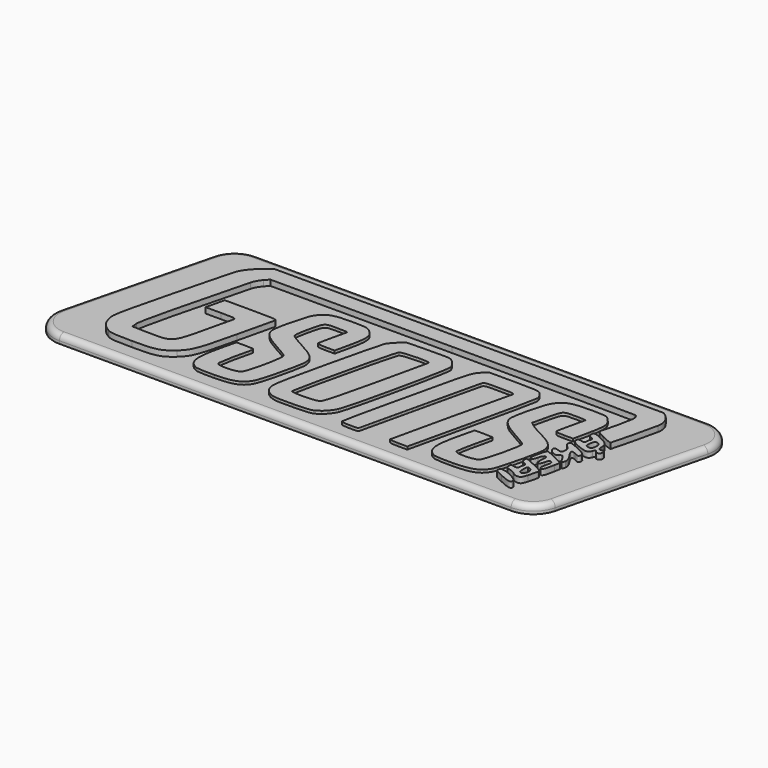
from build123d import *

# Parameters (mm, degrees)
F1_DEPTH = 3
F3_DEPTH = 2
F5_DEPTH = 1
F6_R     = 10
F7_R     = 2


# Not quite as in the source:
# - ends of sketch curves that miss each other by under 0.0002 mm in the source are joined


with BuildPart() as f1:
    # F0 (on Top) → F1 (new body)
    with BuildSketch(Plane.XY):
        Polygon((100, 36), (-82.0483837953, 36), (-100, -36), (82.0483837953, -36), align=None)
    extrude(amount=-F1_DEPTH)

    # F6
    f6_edges = [f1.edges().sort_by_distance(p)[0] for p in [
        (82.048384, -36, -1.5),
        (100, 36, -1.5),
        (-82.048384, 36, -1.5),
        (-100, -36, -1.5),
    ]]
    fillet(f6_edges, radius=F6_R)

    # F7
    f7_edges = [f1.edges().sort_by_distance(p)[0] for p in [
        (90.421013, -2.419219, 0),
        (80.392142, -33.880108, 0),
        (95.080691, 32.156615, 0),
        (-6.482528, -36, 0),
        (6.482528, 36, 0),
        (-95.080691, -32.156615, 0),
        (-80.392142, 33.880108, 0),
        (-90.421013, 2.419219, 0),
    ]]
    fillet(f7_edges, radius=F7_R)


with BuildPart() as f3:
    # F2 (on Top) → F3 (new body)
    with BuildSketch(Plane.XY):
        with BuildLine():
            add(Edge.make_bspline(
                [(-75.795616532, -28.4242405015), (-78.2587663788, -26.9027705255), (-79.2517103888, -25.5686924543), (-79.9744679458, -22.8097125669)],
                knots=[0, 0, 0, 0, 1, 1, 1, 1], degree=3))
            add(Edge.make_bspline(
                [(-66.5146440238, -29.4511190722), (-72.9671780187, -29.4493452772), (-74.3910725204, -29.2918230737), (-75.795616532, -28.4242405015)],
                knots=[0, 0, 0, 0, 1, 1, 1, 1], degree=3))
            add(Edge.make_bspline(
                [(-53.1869458343, -26.1183050096), (-56.5493552568, -29.0705405866), (-58.0804062385, -29.4534059483), (-66.5146440238, -29.4511190722)],
                knots=[0, 0, 0, 0, 1, 1, 1, 1], degree=3))
            add(Edge.make_bspline(
                [(-46.1866547532, -8.0317014306), (-49.2081877021, -21.146458367), (-50.0749640039, -23.3859446112), (-53.1869458343, -26.1183050096)],
                knots=[0, 0, 0, 0, 1, 1, 1, 1], degree=3))
            add(Edge.make_bspline(
                [(-43.1147267619, 4.9727765604), (-43.2790551442, 4.4404873009), (-44.6614235781, -1.4115239207), (-46.1866547532, -8.0317014306)],
                knots=[0, 0, 0, 0, 1, 1, 1, 1], degree=3))
            add(Edge.make_bspline(
                [(-52.2441455618, 5.9405733101), (-43.5197760782, 5.9405733101), (-42.8382534939, 5.8683272922), (-43.1147267619, 4.9727765604)],
                knots=[0, 0, 0, 0, 1, 1, 1, 1], degree=3))
            Line((-52.2441455618, 5.9405733101), (-61.6723430484, 5.9405733101))
            Line((-61.6723430484, 5.9405733101), (-62.0130645506, 4.4197483504))
            add(Edge.make_bspline(
                [(-62.8085644531, 1.1015853731), (-62.5584384271, 2.0901231676), (-62.200462738, 3.583294099), (-62.0130645506, 4.4197483504)],
                knots=[0, 0, 0, 0, 1, 1, 1, 1], degree=3))
            Line((-62.8085644531, 1.1015853731), (-63.2633428535, -0.6957547387))
            Line((-63.2633428535, -0.6957547387), (-57.7403800137, -0.6957547387))
            add(Edge.make_bspline(
                [(-52.5163382668, -1.6635535826), (-52.2454397829, -0.7864905268), (-52.7352228847, -0.6957547387), (-57.7403800137, -0.6957547387)],
                knots=[0, 0, 0, 0, 1, 1, 1, 1], degree=3))
            add(Edge.make_bspline(
                [(-54.5073906057, -10.0972238374), (-53.5767178968, -5.9909912107), (-52.6807441349, -2.195842842), (-52.5163382668, -1.6635535826)],
                knots=[0, 0, 0, 0, 1, 1, 1, 1], degree=3))
            add(Edge.make_bspline(
                [(-65.8975644353, -22.6981373061), (-57.4239911245, -22.9199936065), (-57.410200759, -22.9047331064), (-54.5073906057, -10.0972238374)],
                knots=[0, 0, 0, 0, 1, 1, 1, 1], degree=3))
            Line((-65.8975644353, -22.6981373061), (-71.9244253447, -22.540338667))
            Line((-71.9244253447, -22.540338667), (-72.0935473713, -20.508711031))
            add(Edge.make_bspline(
                [(-62.7643180079, 18.7170547803), (-69.3169468103, -6.5522517558), (-72.2342572659, -18.8184059351), (-72.0935473713, -20.508711031)],
                knots=[0, 0, 0, 0, 1, 1, 1, 1], degree=3))
            add(Edge.make_bspline(
                [(-60.8908869106, 22.1734774279), (-61.637107984, 21.3682897151), (-62.4801527107, 19.8128998378), (-62.7643180079, 18.7170547803)],
                knots=[0, 0, 0, 0, 1, 1, 1, 1], degree=3))
            Line((-60.8908869106, 22.1734774279), (-59.5341201804, 23.6374508991))
            Line((-59.5341201804, 23.6374508991), (5.4277806453, 23.6374508991))
            add(Edge.make_bspline(
                [(71.2644555565, 23.3017701577), (70.7833320084, 23.4863956126), (41.1568291361, 23.6374508991), (5.4277806453, 23.6374508991)],
                knots=[0, 0, 0, 0, 1, 1, 1, 1], degree=3))
            add(Edge.make_bspline(
                [(72.1392317362, 21.3200621788), (72.1392317362, 22.3108617188), (71.7910129663, 23.0997125082), (71.2644555565, 23.3017701577)],
                knots=[0, 0, 0, 0, 1, 1, 1, 1], degree=3))
            add(Edge.make_bspline(
                [(69.6190942774, 9.7772665945), (70.7649155355, 13.6800761474), (72.1392317362, 19.974729829), (72.1392317362, 21.3200621788)],
                knots=[0, 0, 0, 0, 1, 1, 1, 1], degree=3))
            add(Edge.make_bspline(
                [(72.6814852415, 7.3282945418), (70.3223694092, 8.4558480159), (69.4386279213, 9.1625681214), (69.6190942774, 9.7772665945)],
                knots=[0, 0, 0, 0, 1, 1, 1, 1], degree=3))
            add(Edge.make_bspline(
                [(76.2098251162, 5.9802208726), (76.0930708769, 5.8499443266), (74.5053170956, 6.4565800955), (72.6814852415, 7.3282945418)],
                knots=[0, 0, 0, 0, 1, 1, 1, 1], degree=3))
            add(Edge.make_bspline(
                [(80.150160798, 22.3358519134), (79.4319309206, 18.7363340673), (76.4135476618, 6.2075367755), (76.2098251162, 5.9802208726)],
                knots=[0, 0, 0, 0, 1, 1, 1, 1], degree=3))
            add(Edge.make_bspline(
                [(76.4670232856, 29.2734046848), (79.2593031884, 27.7829583192), (80.6967765404, 25.0753326219), (80.150160798, 22.3358519134)],
                knots=[0, 0, 0, 0, 1, 1, 1, 1], degree=3))
            Line((76.4670232856, 29.2734046848), (-62.5478145054, 29.3525971936))
            add(Edge.make_bspline(
                [(-69.849839202, 21.7018573997), (-68.9301925028, 24.02660517), (-65.2045907169, 27.9301246598), (-62.5478145054, 29.3525971936)],
                knots=[0, 0, 0, 0, 1, 1, 1, 1], degree=3))
            add(Edge.make_bspline(
                [(-75.5653436062, -0.1427265287), (-72.7827913036, 10.9593009126), (-70.2108137982, 20.7893624239), (-69.849839202, 21.7018573997)],
                knots=[0, 0, 0, 0, 1, 1, 1, 1], degree=3))
            add(Edge.make_bspline(
                [(-79.9744679458, -22.8097125669), (-80.5884837068, -20.4658383868), (-80.3439806317, -19.2088669923), (-75.5653436062, -0.1427265287)],
                knots=[0, 0, 0, 0, 1, 1, 1, 1], degree=3))
        make_face()
    extrude(amount=F3_DEPTH)


with BuildPart() as f3b:
    # F2 (on Top) → F3, piece 2 (new body)
    with BuildSketch(Plane.XY):
        with BuildLine():
            add(Edge.make_bspline(
                [(70.3418895302, -1.1602418914), (68.5422039045, -0.3665325375), (67.715012339, 0.3276872352), (67.715012339, 1.0443673981)],
                knots=[0, 0, 0, 0, 1, 1, 1, 1], degree=3))
            add(Edge.make_bspline(
                [(75.3841413811, -1.1542315119), (74.8334628735, -2.6428580101), (73.7066716914, -2.644200398), (70.3418895302, -1.1602418914)],
                knots=[0, 0, 0, 0, 1, 1, 1, 1], degree=3))
            add(Edge.make_bspline(
                [(76.228501271, -0.6012012077), (75.9633053179, -0.1721061851), (75.6784279897, -0.3586960078), (75.3841413811, -1.1542315119)],
                knots=[0, 0, 0, 0, 1, 1, 1, 1], degree=3))
            add(Edge.make_bspline(
                [(78.222531575, -0.0782269894), (78.222531575, -1.3307419074), (76.8946230431, -1.6790151267), (76.228501271, -0.6012012077)],
                knots=[0, 0, 0, 0, 1, 1, 1, 1], degree=3))
            add(Edge.make_bspline(
                [(77.1463092547, 0.8108861443), (77.962259107, 1.0242671813), (78.222531575, 0.8091144436), (78.222531575, -0.0782269894)],
                knots=[0, 0, 0, 0, 1, 1, 1, 1], degree=3))
            add(Edge.make_bspline(
                [(75.9019973529, 2.5366901749), (76.0427344723, 0.8560477588), (76.2451983984, 0.5752415727), (77.1463092547, 0.8108861443)],
                knots=[0, 0, 0, 0, 1, 1, 1, 1], degree=3))
            add(Edge.make_bspline(
                [(73.5217970256, 5.735332463), (75.3981725806, 4.7247489317), (75.7594173297, 4.239288277), (75.9019973529, 2.5366901749)],
                knots=[0, 0, 0, 0, 1, 1, 1, 1], degree=3))
            add(Edge.make_bspline(
                [(68.8210645705, 6.5681386025), (68.8210645705, 7.8631010403), (69.9387585092, 7.6650873081), (73.5217970256, 5.735332463)],
                knots=[0, 0, 0, 0, 1, 1, 1, 1], degree=3))
            add(Edge.make_bspline(
                [(69.9671161917, 5.0983411364), (69.3110005496, 5.306585079), (68.8210645705, 5.9349189461), (68.8210645705, 6.5681386025)],
                knots=[0, 0, 0, 0, 1, 1, 1, 1], degree=3))
            add(Edge.make_bspline(
                [(70.7966532711, 3.909787546), (70.9965894871, 4.4307994907), (70.6910423173, 4.8685708207), (69.9671161917, 5.0983411364)],
                knots=[0, 0, 0, 0, 1, 1, 1, 1], degree=3))
            add(Edge.make_bspline(
                [(70.480145012, 2.2407114455), (70.480145012, 2.7050561921), (70.622572158, 3.4561400185), (70.7966532711, 3.909787546)],
                knots=[0, 0, 0, 0, 1, 1, 1, 1], degree=3))
            add(Edge.make_bspline(
                [(69.0975776284, 1.743452018), (70.1200939619, 1.4868150966), (70.480145012, 1.6163167853), (70.480145012, 2.2407114455)],
                knots=[0, 0, 0, 0, 1, 1, 1, 1], degree=3))
            add(Edge.make_bspline(
                [(67.715012339, 1.0443673981), (67.715012339, 1.8840425428), (67.9878144587, 2.021981799), (69.0975776284, 1.743452018)],
                knots=[0, 0, 0, 0, 1, 1, 1, 1], degree=3))
        make_face()
        with BuildLine():
            add(Edge.make_bspline(
                [(74.4812504472, 1.2113700852), (74.7495604889, 2.614942384), (74.0593008652, 3.7284646586), (72.9209370848, 3.7284646586)],
                knots=[0, 0, 0, 0, 1, 1, 1, 1], degree=3))
            add(Edge.make_bspline(
                [(72.375249077, 0.1909479606), (73.6792836276, -0.3503212665), (74.2341044804, -0.0814897668), (74.4812504472, 1.2113700852)],
                knots=[0, 0, 0, 0, 1, 1, 1, 1], degree=3))
            add(Edge.make_bspline(
                [(72.9209370848, 3.7284646586), (72.0812033023, 3.7284646586), (71.5860548374, 0.5185157368), (72.375249077, 0.1909479606)],
                knots=[0, 0, 0, 0, 1, 1, 1, 1], degree=3))
        make_face(mode=Mode.SUBTRACT)
    extrude(amount=F3_DEPTH)


with BuildPart() as f3c:
    # F2 (on Top) → F3, piece 3 (new body)
    with BuildSketch(Plane.XY):
        with BuildLine():
            add(Edge.make_bspline(
                [(72.1772060258, -10.788505435), (70.7775645572, -8.3432882988), (70.598771474, -8.2042579597), (69.7546524182, -8.9048148084)],
                knots=[0, 0, 0, 0, 1, 1, 1, 1], degree=3))
            add(Edge.make_bspline(
                [(73.3956712016, -10.6879540898), (73.0516555089, -12.0034858472), (72.8807219917, -12.0175924382), (72.1772060258, -10.788505435)],
                knots=[0, 0, 0, 0, 1, 1, 1, 1], degree=3))
            add(Edge.make_bspline(
                [(72.3541122268, -7.6756398484), (73.1051792995, -8.7809339764), (73.5545295104, -10.080497391), (73.3956712016, -10.6879540898)],
                knots=[0, 0, 0, 0, 1, 1, 1, 1], degree=3))
            add(Edge.make_bspline(
                [(72.6321708108, -5.3654363587), (70.65545752, -4.3432404392), (70.5703237406, -5.0505573942), (72.3541122268, -7.6756398484)],
                knots=[0, 0, 0, 0, 1, 1, 1, 1], degree=3))
            add(Edge.make_bspline(
                [(74.5014218671, -5.1588342759), (74.2513335369, -6.1151777972), (74.1118320007, -6.1305974572), (72.6321708108, -5.3654363587)],
                knots=[0, 0, 0, 0, 1, 1, 1, 1], degree=3))
            add(Edge.make_bspline(
                [(71.1050904492, -2.4172007207), (74.0419880404, -3.7854227735), (74.717900239, -4.3310353898), (74.5014218671, -5.1588342759)],
                knots=[0, 0, 0, 0, 1, 1, 1, 1], degree=3))
            add(Edge.make_bspline(
                [(67.2419850024, -1.6238829838), (67.4125750693, -0.8297129039), (67.9221400682, -0.934354239), (71.1050904492, -2.4172007207)],
                knots=[0, 0, 0, 0, 1, 1, 1, 1], degree=3))
            add(Edge.make_bspline(
                [(68.2609893476, -3.4555974401), (67.5924550469, -2.9513224129), (67.1338965995, -2.1270522687), (67.2419850024, -1.6238829838)],
                knots=[0, 0, 0, 0, 1, 1, 1, 1], degree=3))
            add(Edge.make_bspline(
                [(69.2739121103, -5.7140278979), (69.4095184179, -4.816060449), (69.0745874033, -4.0692969756), (68.2609893476, -3.4555974401)],
                knots=[0, 0, 0, 0, 1, 1, 1, 1], degree=3))
            add(Edge.make_bspline(
                [(67.0237223645, -6.4843721633), (68.7801709537, -7.1679596375), (69.0692974317, -7.0689810432), (69.2739121103, -5.7140278979)],
                knots=[0, 0, 0, 0, 1, 1, 1, 1], degree=3))
            add(Edge.make_bspline(
                [(67.5003894361, -8.9187643338), (65.8372378525, -8.1609832274), (65.383992413, -5.8462059855), (67.0237223645, -6.4843721633)],
                knots=[0, 0, 0, 0, 1, 1, 1, 1], degree=3))
            add(Edge.make_bspline(
                [(69.7546524182, -8.9048148084), (69.1252630698, -9.4271628583), (68.6230613093, -9.4302664759), (67.5003894361, -8.9187643338)],
                knots=[0, 0, 0, 0, 1, 1, 1, 1], degree=3))
        make_face()
    extrude(amount=F3_DEPTH)


with BuildPart() as f3d:
    # F2 (on Top) → F3, piece 4 (new body)
    with BuildSketch(Plane.XY):
        with BuildLine():
            add(Edge.make_bspline(
                [(70.3506789249, -18.0788235038), (70.1780867942, -17.9062313732), (70.2822443671, -16.8763580839), (70.5821392671, -15.7902175904)],
                knots=[0, 0, 0, 0, 1, 1, 1, 1], degree=3))
            add(Edge.make_bspline(
                [(72.4411182289, -14.4188395648), (71.7683410609, -18.2187920485), (71.3038664734, -19.0320110524), (70.3506789249, -18.0788235038)],
                knots=[0, 0, 0, 0, 1, 1, 1, 1], degree=3))
            Line((72.4411182289, -14.4188395648), (72.8019734552, -12.3806403013))
            Line((72.8019734552, -12.3806403013), (69.4447220692, -10.6859038593))
            add(Edge.make_bspline(
                [(65.8211794588, -8.9911653232), (65.9676358626, -8.9911653232), (67.598230875, -9.7537966173), (69.4447220692, -10.6859038593)],
                knots=[0, 0, 0, 0, 1, 1, 1, 1], degree=3))
            add(Edge.make_bspline(
                [(64.3999299429, -14.4292708192), (64.4034754386, -12.9248874934), (65.4316063461, -8.9911653232), (65.8211794588, -8.9911653232)],
                knots=[0, 0, 0, 0, 1, 1, 1, 1], degree=3))
            add(Edge.make_bspline(
                [(66.0559256148, -13.6918998725), (65.7109800933, -15.6477548429), (64.3956158726, -16.2334506172), (64.3999299429, -14.4292708192)],
                knots=[0, 0, 0, 0, 1, 1, 1, 1], degree=3))
            add(Edge.make_bspline(
                [(67.0775477211, -11.8761600415), (66.667738268, -12.0125097933), (66.2080091579, -12.8295884241), (66.0559256148, -13.6918998725)],
                knots=[0, 0, 0, 0, 1, 1, 1, 1], degree=3))
            add(Edge.make_bspline(
                [(67.6305717427, -13.9923392669), (67.7763852244, -12.197675554), (67.6431600323, -11.6879681489), (67.0775477211, -11.8761600415)],
                knots=[0, 0, 0, 0, 1, 1, 1, 1], degree=3))
            add(Edge.make_bspline(
                [(69.1748078635, -14.8390446707), (68.5110965258, -17.553608482), (67.3911198994, -16.9395278005), (67.6305717427, -13.9923392669)],
                knots=[0, 0, 0, 0, 1, 1, 1, 1], degree=3))
            add(Edge.make_bspline(
                [(70.3890071358, -13.3542359154), (69.8480834531, -13.0163960446), (69.5233575184, -13.4134873672), (69.1748078635, -14.8390446707)],
                knots=[0, 0, 0, 0, 1, 1, 1, 1], degree=3))
            add(Edge.make_bspline(
                [(70.5821392671, -15.7902175904), (71.0000156128, -14.276785188), (70.9548916941, -13.7076734538), (70.3890071358, -13.3542359154)],
                knots=[0, 0, 0, 0, 1, 1, 1, 1], degree=3))
        make_face()
    extrude(amount=F3_DEPTH)


with BuildPart() as f3e:
    # F2 (on Top) → F3, piece 5 (new body)
    with BuildSketch(Plane.XY):
        with BuildLine():
            add(Edge.make_bspline(
                [(66.6642681639, -25.3721216319), (66.3160389229, -24.9525364118), (65.2901195, -24.4610339645), (64.3844390798, -24.2798932732)],
                knots=[0, 0, 0, 0, 1, 1, 1, 1], degree=3))
            add(Edge.make_bspline(
                [(68.5909508046, -26.1350188906), (67.8795019754, -26.1350188906), (67.0124994991, -25.7917131347), (66.6642681639, -25.3721216319)],
                knots=[0, 0, 0, 0, 1, 1, 1, 1], degree=3))
            add(Edge.make_bspline(
                [(70.4917532119, -23.7846505689), (69.9951262354, -25.7068055299), (69.6488215724, -26.1350188906), (68.5909508046, -26.1350188906)],
                knots=[0, 0, 0, 0, 1, 1, 1, 1], degree=3))
            add(Edge.make_bspline(
                [(71.3736559844, -20.4860684446), (71.2225986036, -21.007589282), (70.8257397383, -22.4919498767), (70.4917532119, -23.7846505689)],
                knots=[0, 0, 0, 0, 1, 1, 1, 1], degree=3))
            add(Edge.make_bspline(
                [(67.9460810641, -17.8591912533), (70.8015600025, -19.1539296108), (71.5854873068, -19.7547267253), (71.3736559844, -20.4860684446)],
                knots=[0, 0, 0, 0, 1, 1, 1, 1], degree=3))
            add(Edge.make_bspline(
                [(64.0438390418, -16.1805236762), (64.1538541169, -16.1805236762), (65.9098629222, -16.9359215728), (67.9460810641, -17.8591912533)],
                knots=[0, 0, 0, 0, 1, 1, 1, 1], degree=3))
            add(Edge.make_bspline(
                [(63.8438148691, -17.2493094607), (63.8438148691, -16.6614817817), (63.9338302493, -16.1805236762), (64.0438390418, -16.1805236762)],
                knots=[0, 0, 0, 0, 1, 1, 1, 1], degree=3))
            add(Edge.make_bspline(
                [(64.9898685844, -18.681842574), (64.3513003185, -18.4791650386), (63.8438148691, -17.8448291688), (63.8438148691, -17.2493094607)],
                knots=[0, 0, 0, 0, 1, 1, 1, 1], degree=3))
            add(Edge.make_bspline(
                [(65.8194056639, -19.8703961644), (66.0193397857, -19.3493842198), (65.7137947101, -18.9116066071), (64.9898685844, -18.681842574)],
                knots=[0, 0, 0, 0, 1, 1, 1, 1], degree=3))
            add(Edge.make_bspline(
                [(65.5029015932, -21.5394659823), (65.5029015932, -21.0751212357), (65.6453287392, -20.3240374093), (65.8194056639, -19.8703961644)],
                knots=[0, 0, 0, 0, 1, 1, 1, 1], degree=3))
            add(Edge.make_bspline(
                [(64.1203300212, -22.0367316924), (65.1428463547, -22.2933623312), (65.5029015932, -22.1638627367), (65.5029015932, -21.5394659823)],
                knots=[0, 0, 0, 0, 1, 1, 1, 1], degree=3))
            add(Edge.make_bspline(
                [(62.7377626375, -22.8201438213), (62.7377626375, -21.8905161226), (62.9833379476, -21.7513622252), (64.1203300212, -22.0367316924)],
                knots=[0, 0, 0, 0, 1, 1, 1, 1], degree=3))
            add(Edge.make_bspline(
                [(64.3844390798, -24.2798932732), (63.2020319925, -24.0434152065), (62.7377626375, -23.6318508063), (62.7377626375, -22.8201438213)],
                knots=[0, 0, 0, 0, 1, 1, 1, 1], degree=3))
        make_face()
        with BuildLine():
            add(Edge.make_bspline(
                [(69.2842198064, -22.2830504467), (69.4532015209, -21.1271623264), (68.6504556557, -20.0821039285), (67.5767526687, -20.0601838441)],
                knots=[0, 0, 0, 0, 1, 1, 1, 1], degree=3))
            add(Edge.make_bspline(
                [(67.5421772801, -23.5657491973), (68.2163198722, -24.2398813183), (69.0924530993, -23.5947686497), (69.2842198064, -22.2830504467)],
                knots=[0, 0, 0, 0, 1, 1, 1, 1], degree=3))
            add(Edge.make_bspline(
                [(67.5767526687, -20.0601838441), (67.0567501327, -20.049545263), (67.0271568671, -23.0507120306), (67.5421772801, -23.5657491973)],
                knots=[0, 0, 0, 0, 1, 1, 1, 1], degree=3))
        make_face(mode=Mode.SUBTRACT)
    extrude(amount=F3_DEPTH)


with BuildPart() as f3f:
    # F2 (on Top) → F3, piece 6 (new body)
    with BuildSketch(Plane.XY):
        with BuildLine():
            add(Edge.make_bspline(
                [(64.811613713, -28.4448098211), (61.4677820175, -26.9169378486), (61.3825079261, -26.8309119362), (62.0964760885, -25.7058777954)],
                knots=[0, 0, 0, 0, 1, 1, 1, 1], degree=3))
            add(Edge.make_bspline(
                [(69.3558124312, -29.0384300819), (69.3795712309, -30.2966894148), (68.6583466347, -30.2024688631), (64.811613713, -28.4448098211)],
                knots=[0, 0, 0, 0, 1, 1, 1, 1], degree=3))
            add(Edge.make_bspline(
                [(62.0964760885, -25.7058777954), (62.7472787227, -24.6803772142), (69.33057512, -27.7025844983), (69.3558124312, -29.0384300819)],
                knots=[0, 0, 0, 0, 1, 1, 1, 1], degree=3))
        make_face()
    extrude(amount=F3_DEPTH)


with BuildPart() as f5:
    # F4 (on Top) → F5 (new body)
    with BuildSketch(Plane.XY):
        with BuildLine():
            add(Edge.make_bspline(
                [(-43.7196340114, -29.2730058155), (-47.3438458097, -27.6913644979), (-47.7971835336, -24.6050915181), (-45.6983651989, -15.8019934908)],
                knots=[0, 0, 0, 0, 1, 1, 1, 1], degree=3))
            add(Edge.make_bspline(
                [(-36.8068525567, -29.6169116317), (-40.0005574924, -29.6932364868), (-43.1113094612, -29.5384779271), (-43.7196340114, -29.2730058155)],
                knots=[0, 0, 0, 0, 1, 1, 1, 1], degree=3))
            add(Edge.make_bspline(
                [(-26.1661466294, -25.4411885684), (-27.9927956322, -28.5448370441), (-30.3302427488, -29.4621216592), (-36.8068525567, -29.6169116317)],
                knots=[0, 0, 0, 0, 1, 1, 1, 1], degree=3))
            add(Edge.make_bspline(
                [(-21.8752389181, -7.9434317753), (-21.8752389181, -10.3860281805), (-25.1393170205, -23.6964998865), (-26.1661466294, -25.4411885684)],
                knots=[0, 0, 0, 0, 1, 1, 1, 1], degree=3))
            add(Edge.make_bspline(
                [(-28.4696259814, -0.7543742817), (-23.2797033701, -3.5105589121), (-21.8752389181, -5.0416799859), (-21.8752389181, -7.9434317753)],
                knots=[0, 0, 0, 0, 1, 1, 1, 1], degree=3))
            add(Edge.make_bspline(
                [(-34.0794483819, 2.6314411897), (-33.7475569346, 2.231534634), (-31.2231363309, 0.707921232), (-28.4696259814, -0.7543742817)],
                knots=[0, 0, 0, 0, 1, 1, 1, 1], degree=3))
            add(Edge.make_bspline(
                [(-33.7372786493, 7.672967391), (-34.4277813161, 4.5224802578), (-34.5200911248, 3.162385413), (-34.0794483819, 2.6314411897)],
                knots=[0, 0, 0, 0, 1, 1, 1, 1], degree=3))
            add(Edge.make_bspline(
                [(-27.9390377704, 13.9229648801), (-32.4400262632, 13.9229648801), (-32.3449877247, 14.0254126634), (-33.7372786493, 7.672967391)],
                knots=[0, 0, 0, 0, 1, 1, 1, 1], degree=3))
            add(Edge.make_bspline(
                [(-24.0873319993, 13.6814900936), (-24.0873319993, 13.8143057287), (-25.8206010622, 13.9229648801), (-27.9390377704, 13.9229648801)],
                knots=[0, 0, 0, 0, 1, 1, 1, 1], degree=3))
            add(Edge.make_bspline(
                [(-25.189504288, 8.8425432847), (-24.5833137176, 11.3711459862), (-24.0873319993, 13.5486744586), (-24.0873319993, 13.6814900936)],
                knots=[0, 0, 0, 0, 1, 1, 1, 1], degree=3))
            add(Edge.make_bspline(
                [(-26.2955487344, 3.5537979333), (-26.2933623999, 3.9340002537), (-25.7956990468, 6.3139363948), (-25.189504288, 8.8425432847)],
                knots=[0, 0, 0, 0, 1, 1, 1, 1], degree=3))
            add(Edge.make_bspline(
                [(-23.1128215435, 2.8625162277), (-25.2954891586, 2.8625162277), (-26.2982020734, 3.0803036291), (-26.2955487344, 3.5537979333)],
                knots=[0, 0, 0, 0, 1, 1, 1, 1], degree=3))
            Line((-23.1128215435, 2.8625162277), (-19.9262159124, 2.8625162277))
            Line((-19.9262159124, 2.8625162277), (-18.7311181231, 8.2544842128))
            add(Edge.make_bspline(
                [(-19.7712123325, 18.0766968523), (-17.522567256, 16.1845897472), (-17.3450343782, 14.5080941799), (-18.7311181231, 8.2544842128)],
                knots=[0, 0, 0, 0, 1, 1, 1, 1], degree=3))
            add(Edge.make_bspline(
                [(-27.2443697593, 19.4531933946), (-21.8316211251, 19.4531933946), (-21.2881075724, 19.3530848217), (-19.7712123325, 18.0766968523)],
                knots=[0, 0, 0, 0, 1, 1, 1, 1], degree=3))
            add(Edge.make_bspline(
                [(-37.8213913634, 15.4159046786), (-35.8472255105, 18.679674935), (-33.8207405045, 19.4531933946), (-27.2443697593, 19.4531933946)],
                knots=[0, 0, 0, 0, 1, 1, 1, 1], degree=3))
            add(Edge.make_bspline(
                [(-41.2310324364, 1.7571356396), (-41.2310324364, 4.4197413821), (-38.9531231464, 13.544879786), (-37.8213913634, 15.4159046786)],
                knots=[0, 0, 0, 0, 1, 1, 1, 1], degree=3))
            add(Edge.make_bspline(
                [(-34.1706482698, -5.2992611889), (-39.1403395597, -2.6545984679), (-41.2310324364, -0.5650867144), (-41.2310324364, 1.7571356396)],
                knots=[0, 0, 0, 0, 1, 1, 1, 1], degree=3))
            add(Edge.make_bspline(
                [(-29.1101822126, -8.4194453903), (-29.4594407789, -7.9986157805), (-31.7366506093, -6.5945324711), (-34.1706482698, -5.2992611889)],
                knots=[0, 0, 0, 0, 1, 1, 1, 1], degree=3))
            add(Edge.make_bspline(
                [(-32.2662713044, -23.2678003101), (-30.9570631866, -21.7609404294), (-28.322898641, -9.3680674671), (-29.1101822126, -8.4194453903)],
                knots=[0, 0, 0, 0, 1, 1, 1, 1], degree=3))
            add(Edge.make_bspline(
                [(-40.451480615, -23.4752193759), (-39.9887567308, -24.681062455), (-33.3479498481, -24.5127796152), (-32.2662713044, -23.2678003101)],
                knots=[0, 0, 0, 0, 1, 1, 1, 1], degree=3))
            add(Edge.make_bspline(
                [(-38.1088063997, -11.377813611), (-39.2735426199, -15.5458593731), (-40.6891376927, -22.8558940447), (-40.451480615, -23.4752193759)],
                knots=[0, 0, 0, 0, 1, 1, 1, 1], degree=3))
            add(Edge.make_bspline(
                [(-41.1255920553, -10.4100255057), (-38.2605535139, -10.4100255057), (-37.8730969188, -10.5343177868), (-38.1088063997, -11.377813611)],
                knots=[0, 0, 0, 0, 1, 1, 1, 1], degree=3))
            Line((-41.1255920553, -10.4100255057), (-44.4128214301, -10.4100255057))
            Line((-44.4128214301, -10.4100255057), (-45.6983651989, -15.8019934908))
        make_face()
    extrude(amount=F5_DEPTH)


with BuildPart() as f5b:
    # F4 (on Top) → F5, piece 2 (new body)
    with BuildSketch(Plane.XY):
        with BuildLine():
            add(Edge.make_bspline(
                [(-17.4510590383, -28.8265496006), (-18.8028043469, -28.1307570093), (-19.5861319933, -27.2190806356), (-20.048014013, -25.8041033489)],
                knots=[0, 0, 0, 0, 1, 1, 1, 1], degree=3))
            add(Edge.make_bspline(
                [(-8.8356067332, -29.6560792705), (-14.4087116974, -29.7952256425), (-15.8361787343, -29.6578530496), (-17.4510590383, -28.8265496006)],
                knots=[0, 0, 0, 0, 1, 1, 1, 1], degree=3))
            add(Edge.make_bspline(
                [(-0.0597876272, -27.8902204201), (-2.0659715536, -29.4208221347), (-2.4418116758, -29.4964496245), (-8.8356067332, -29.6560792705)],
                knots=[0, 0, 0, 0, 1, 1, 1, 1], degree=3))
            add(Edge.make_bspline(
                [(2.9942557659, -24.0190596223), (2.4673072575, -25.2686985005), (1.0929865788, -27.0107191842), (-0.0597876272, -27.8902204201)],
                knots=[0, 0, 0, 0, 1, 1, 1, 1], degree=3))
            add(Edge.make_bspline(
                [(11.6457972503, 15.2506961099), (12.0731628275, 13.547941492), (4.6747449539, -20.0338303798), (2.9942557659, -24.0190596223)],
                knots=[0, 0, 0, 0, 1, 1, 1, 1], degree=3))
            add(Edge.make_bspline(
                [(9.7785775012, 18.156562983), (10.5941179808, 17.4007446188), (11.4343678103, 16.0931029553), (11.6457972503, 15.2506961099)],
                knots=[0, 0, 0, 0, 1, 1, 1, 1], degree=3))
            add(Edge.make_bspline(
                [(0.4342276466, 19.3537235497), (8.1552450457, 19.5276041599), (8.3222860307, 19.5062015363), (9.7785775012, 18.156562983)],
                knots=[0, 0, 0, 0, 1, 1, 1, 1], degree=3))
            Line((0.4342276466, 19.3537235497), (-7.4273308551, 19.1766807124))
            Line((-7.4273308551, 19.1766807124), (-9.1686562676, 17.5176150899))
            add(Edge.make_bspline(
                [(-11.5005160849, 14.7680795133), (-11.1757176598, 15.3678367315), (-10.1263796949, 16.6051282645), (-9.1686562676, 17.5176150899)],
                knots=[0, 0, 0, 0, 1, 1, 1, 1], degree=3))
            add(Edge.make_bspline(
                [(-16.4002258217, -5.0501782096), (-14.030182635, 5.2501045397), (-11.8253166041, 14.1683181067), (-11.5005160849, 14.7680795133)],
                knots=[0, 0, 0, 0, 1, 1, 1, 1], degree=3))
            add(Edge.make_bspline(
                [(-20.048014013, -25.8041033489), (-20.6480832655, -23.9657834242), (-20.3099511316, -22.0419849392), (-16.4002258217, -5.0501782096)],
                knots=[0, 0, 0, 0, 1, 1, 1, 1], degree=3))
        make_face()
        with BuildLine():
            add(Edge.make_bspline(
                [(-3.985248682, -23.5352975036), (-3.2954433805, -23.0309034233), (-1.8736264687, -17.836828033), (1.0976545287, -4.9667770859)],
                knots=[0, 0, 0, 0, 1, 1, 1, 1], degree=3))
            add(Edge.make_bspline(
                [(-13.8164097962, -23.7472881866), (-13.3420505914, -24.514825639), (-5.0812200737, -24.3366959169), (-3.985248682, -23.5352975036)],
                knots=[0, 0, 0, 0, 1, 1, 1, 1], degree=3))
            add(Edge.make_bspline(
                [(-5.22164809, 13.1692469886), (-6.0072814397, 12.2226164867), (-14.2269904392, -23.0829670853), (-13.8164097962, -23.7472881866)],
                knots=[0, 0, 0, 0, 1, 1, 1, 1], degree=3))
            add(Edge.make_bspline(
                [(5.2228636308, 13.4122170268), (5.2228636308, 14.2678947553), (-4.4975211057, 14.0417682886), (-5.22164809, 13.1692469886)],
                knots=[0, 0, 0, 0, 1, 1, 1, 1], degree=3))
            add(Edge.make_bspline(
                [(1.0976545287, -4.9667770859), (3.3665190113, 4.8607547967), (5.2228636308, 13.1313023568), (5.2228636308, 13.4122170268)],
                knots=[0, 0, 0, 0, 1, 1, 1, 1], degree=3))
        make_face(mode=Mode.SUBTRACT)
    extrude(amount=F5_DEPTH)


with BuildPart() as f5c:
    # F4 (on Top) → F5, piece 3 (new body)
    with BuildSketch(Plane.XY):
        with BuildLine():
            add(Edge.make_bspline(
                [(8.3805443072, -29.3510437181), (8.2563923369, -29.1229256766), (9.8581713872, -21.5949025615), (11.9400581942, -12.6221143985)],
                knots=[0, 0, 0, 0, 1, 1, 1, 1], degree=3))
            add(Edge.make_bspline(
                [(14.6242424722, -29.5023238279), (14.6242424722, -29.941976019), (8.6230075514, -29.7965722068), (8.3805443072, -29.3510437181)],
                knots=[0, 0, 0, 0, 1, 1, 1, 1], degree=3))
            add(Edge.make_bspline(
                [(24.3868544594, 12.6786640925), (23.6574166088, 9.7667743285), (14.6242424722, -29.2625683716), (14.6242424722, -29.5023238279)],
                knots=[0, 0, 0, 0, 1, 1, 1, 1], degree=3))
            add(Edge.make_bspline(
                [(30.2060958773, 13.9229648801), (24.9556071921, 13.9229648801), (24.6840053858, 13.8648678562), (24.3868544594, 12.6786640925)],
                knots=[0, 0, 0, 0, 1, 1, 1, 1], degree=3))
            add(Edge.make_bspline(
                [(35.4157143471, 12.9551767748), (35.6856428955, 13.8320414253), (35.196178297, 13.9229648801), (30.2060958773, 13.9229648801)],
                knots=[0, 0, 0, 0, 1, 1, 1, 1], degree=3))
            add(Edge.make_bspline(
                [(25.6846911245, -29.32507576), (25.6846911245, -28.8238418127), (34.9585442553, 11.4700441172), (35.4157143471, 12.9551767748)],
                knots=[0, 0, 0, 0, 1, 1, 1, 1], degree=3))
            add(Edge.make_bspline(
                [(28.9052980273, -29.7658106473), (27.1339670579, -29.7658106473), (25.6846911245, -29.5674845552), (25.6846911245, -29.32507576)],
                knots=[0, 0, 0, 0, 1, 1, 1, 1], degree=3))
            Line((28.9052980273, -29.7658106473), (32.1259049301, -29.7658106473))
            Line((32.1259049301, -29.7658106473), (37.2024376143, -7.7831634012))
            add(Edge.make_bspline(
                [(42.2771713891, 15.5463915742), (42.2783546066, 14.8055864593), (39.9945313236, 4.3072875581), (37.2024376143, -7.7831634012)],
                knots=[0, 0, 0, 0, 1, 1, 1, 1], degree=3))
            add(Edge.make_bspline(
                [(41.0729240829, 18.1732473961), (41.7342714341, 17.4692811806), (42.2761850256, 16.287196689), (42.2771713891, 15.5463915742)],
                knots=[0, 0, 0, 0, 1, 1, 1, 1], degree=3))
            add(Edge.make_bspline(
                [(30.8845464797, 19.4531933946), (39.5623951811, 19.4531933946), (39.911704008, 19.4093389582), (41.0729240829, 18.1732473961)],
                knots=[0, 0, 0, 0, 1, 1, 1, 1], degree=3))
            Line((30.8845464797, 19.4531933946), (21.8986193677, 19.4531933946))
            Line((21.8986193677, 19.4531933946), (20.2545669945, 17.8091452098))
            add(Edge.make_bspline(
                [(17.1679044953, 9.9285735556), (18.3512811023, 15.0444037184), (18.9059483119, 16.4605286214), (20.2545669945, 17.8091452098)],
                knots=[0, 0, 0, 0, 1, 1, 1, 1], degree=3))
            add(Edge.make_bspline(
                [(11.9400581942, -12.6221143985), (14.0219387187, -3.6493262356), (16.374468193, 6.4984848097), (17.1679044953, 9.9285735556)],
                knots=[0, 0, 0, 0, 1, 1, 1, 1], degree=3))
        make_face()
    extrude(amount=F5_DEPTH)


with BuildPart() as f5d:
    # F4 (on Top) → F5, piece 4 (new body)
    with BuildSketch(Plane.XY):
        with BuildLine():
            add(Edge.make_bspline(
                [(41.4458344331, -29.2730058155), (37.8216268231, -27.6913644979), (37.3682849109, -24.6050915181), (39.4671053398, -15.8019934908)],
                knots=[0, 0, 0, 0, 1, 1, 1, 1], degree=3))
            add(Edge.make_bspline(
                [(48.3586158878, -29.6169116317), (45.1649130463, -29.6932364868), (42.0541589833, -29.5384779271), (41.4458344331, -29.2730058155)],
                knots=[0, 0, 0, 0, 1, 1, 1, 1], degree=3))
            add(Edge.make_bspline(
                [(58.9993239093, -25.4411885684), (57.1726728123, -28.5448370441), (54.8352319783, -29.4621216592), (48.3586158878, -29.6169116317)],
                knots=[0, 0, 0, 0, 1, 1, 1, 1], degree=3))
            add(Edge.make_bspline(
                [(63.2902274322, -7.9434317753), (63.2902274322, -10.3860281805), (60.0261493298, -23.6964998865), (58.9993239093, -25.4411885684)],
                knots=[0, 0, 0, 0, 1, 1, 1, 1], degree=3))
            add(Edge.make_bspline(
                [(57.3303569557, -1.0702430799), (61.801300102, -3.3186410419), (63.2902274322, -5.0357324858), (63.2902274322, -7.9434317753)],
                knots=[0, 0, 0, 0, 1, 1, 1, 1], degree=3))
            add(Edge.make_bspline(
                [(51.7324169902, 2.1526506785), (52.4622045706, 1.5613874957), (54.9812787068, 0.1110833149), (57.3303569557, -1.0702430799)],
                knots=[0, 0, 0, 0, 1, 1, 1, 1], degree=3))
            Line((51.7324169902, 2.1526506785), (50.4055255306, 3.2276696975))
            Line((50.4055255306, 3.2276696975), (51.3553706145, 7.3310154542))
            add(Edge.make_bspline(
                [(57.1951183426, 13.9229648801), (52.722906117, 13.9229648801), (52.9372904593, 14.1649674024), (51.3553706145, 7.3310154542)],
                knots=[0, 0, 0, 0, 1, 1, 1, 1], degree=3))
            add(Edge.make_bspline(
                [(61.0781364452, 13.6814900936), (61.0781364452, 13.8143057287), (59.3307776708, 13.9229648801), (57.1951183426, 13.9229648801)],
                knots=[0, 0, 0, 0, 1, 1, 1, 1], degree=3))
            add(Edge.make_bspline(
                [(59.9759662507, 8.8425432847), (60.5821589153, 11.3711459862), (61.0781364452, 13.5486744586), (61.0781364452, 13.6814900936)],
                knots=[0, 0, 0, 0, 1, 1, 1, 1], degree=3))
            add(Edge.make_bspline(
                [(58.8699238985, 3.5537979333), (58.8722882392, 3.9340002537), (59.369773586, 6.3139363948), (59.9759662507, 8.8425432847)],
                knots=[0, 0, 0, 0, 1, 1, 1, 1], degree=3))
            add(Edge.make_bspline(
                [(62.0883968214, 2.8625162277), (59.8771288512, 2.8625162277), (58.8672579944, 3.079421975), (58.8699238985, 3.5537979333)],
                knots=[0, 0, 0, 0, 1, 1, 1, 1], degree=3))
            Line((62.0883968214, 2.8625162277), (65.3107481846, 2.8625162277))
            Line((65.3107481846, 2.8625162277), (66.4827659041, 8.3087698105))
            add(Edge.make_bspline(
                [(65.6003453671, 17.9323799248), (67.6603227565, 15.7120922775), (67.7845019513, 14.3578192814), (66.4827659041, 8.3087698105)],
                knots=[0, 0, 0, 0, 1, 1, 1, 1], degree=3))
            add(Edge.make_bspline(
                [(58.1365720064, 19.4531933946), (64.0288462125, 19.4531933946), (64.2267513724, 19.4128844221), (65.6003453671, 17.9323799248)],
                knots=[0, 0, 0, 0, 1, 1, 1, 1], degree=3))
            add(Edge.make_bspline(
                [(47.3440812695, 15.4159046786), (49.3360561156, 18.7091255315), (51.3251032839, 19.4531933946), (58.1365720064, 19.4531933946)],
                knots=[0, 0, 0, 0, 1, 1, 1, 1], degree=3))
            add(Edge.make_bspline(
                [(43.9344360081, 1.7571356396), (43.9344360081, 4.4197413821), (46.2123473922, 13.544879786), (47.3440812695, 15.4159046786)],
                knots=[0, 0, 0, 0, 1, 1, 1, 1], degree=3))
            add(Edge.make_bspline(
                [(50.9948201747, -5.2992611889), (46.0251351674, -2.6545984679), (43.9344360081, -0.5650867144), (43.9344360081, 1.7571356396)],
                knots=[0, 0, 0, 0, 1, 1, 1, 1], degree=3))
            add(Edge.make_bspline(
                [(56.0849881312, -8.4552330062), (55.7193948815, -8.0147221972), (53.4288241177, -6.5945324711), (50.9948201747, -5.2992611889)],
                knots=[0, 0, 0, 0, 1, 1, 1, 1], degree=3))
            add(Edge.make_bspline(
                [(55.2502271742, -15.7780862158), (56.4349294035, -10.6252579951), (56.6101628605, -9.0880281686), (56.0849881312, -8.4552330062)],
                knots=[0, 0, 0, 0, 1, 1, 1, 1], degree=3))
            add(Edge.make_bspline(
                [(52.9045582669, -23.2678003101), (53.3699627145, -22.7355137109), (54.42551833, -19.3651407978), (55.2502271742, -15.7780862158)],
                knots=[0, 0, 0, 0, 1, 1, 1, 1], degree=3))
            add(Edge.make_bspline(
                [(44.7234033086, -23.4997486254), (45.1771703413, -24.6822561434), (51.8327894311, -24.4935528552), (52.9045582669, -23.2678003101)],
                knots=[0, 0, 0, 0, 1, 1, 1, 1], degree=3))
            add(Edge.make_bspline(
                [(45.8467981205, -16.8144402015), (45.0736272966, -20.0866500444), (44.5680939768, -23.0950296207), (44.7234033086, -23.4997486254)],
                knots=[0, 0, 0, 0, 1, 1, 1, 1], degree=3))
            add(Edge.make_bspline(
                [(47.2525735356, -10.6374985367), (47.2525735356, -10.7626138344), (46.6199731329, -13.5422366412), (45.8467981205, -16.8144402015)],
                knots=[0, 0, 0, 0, 1, 1, 1, 1], degree=3))
            add(Edge.make_bspline(
                [(44.002610275, -10.4100255057), (45.7900895448, -10.4100255057), (47.2525735356, -10.5123895215), (47.2525735356, -10.6374985367)],
                knots=[0, 0, 0, 0, 1, 1, 1, 1], degree=3))
            Line((44.002610275, -10.4100255057), (40.7526470144, -10.4100255057))
            Line((40.7526470144, -10.4100255057), (39.4671053398, -15.8019934908))
        make_face()
    extrude(amount=F5_DEPTH)


solid = Compound([f1.part, f3.part, f3b.part, f3c.part, f3d.part, f3e.part, f3f.part, f5.part, f5b.part, f5c.part, f5d.part])
